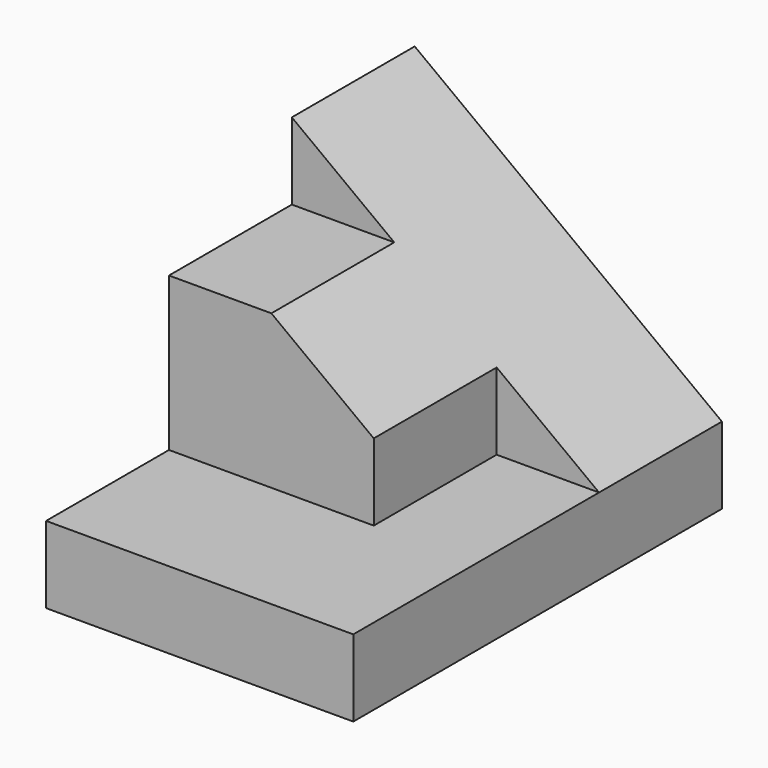
from build123d import *

# Parameters (mm, degrees)
F0_W     = 25.4
F0_H     = 6.35
F1_DEPTH = 38.1
F2_W     = 25.4
F2_H     = 6.35
F3_DEPTH = 25.401
F5_DEPTH = 25.4
F6_W     = 12.7
F6_H     = 6.35
F7_DEPTH = 25.401
F8_W     = 12.7
F8_H     = 6.35
F9_DEPTH = 25.401


# Not quite as in the source:
# - a feature names something its author has since deleted; it is built from what else it names


with BuildPart() as f1:
    # F0 (on Front) → F1 (new body)
    with BuildSketch(Plane.XZ):
        Polygon((25.4, 6.35), (0, 25.4), (0, 6.35), align=None)
        with Locations((12.7, 3.175)):
            Rectangle(F0_W, F0_H)
    extrude(amount=F1_DEPTH)

    # F2 (on face) → F3 (cut, through all)
    with BuildSketch(Plane(origin=(0, 0, 0), x_dir=(0, -1, 0), z_dir=(-1, 0, 0))):
        with Locations((25.4, 22.225)):
            Rectangle(F2_W, F2_H)
    extrude(amount=-F3_DEPTH, mode=Mode.SUBTRACT)

    # F4 (on face) → F5 (cut)
    with BuildSketch(Plane.XZ.offset(38.1)):
        Polygon((16.9333333333, 6.35), (25.4, 6.35), (16.9333333333, 12.7), align=None)
    extrude(amount=-F5_DEPTH, mode=Mode.SUBTRACT)

    # F6 (on face) → F7 (cut, through all)
    with BuildSketch(Plane(origin=(0, 0, 0), x_dir=(0, -1, 0), z_dir=(-1, 0, 0))):
        with Locations((31.75, 15.875)):
            Rectangle(F6_W, F6_H)
    extrude(amount=-F7_DEPTH, mode=Mode.SUBTRACT)

    # F8 (on face) → F9 (cut, through all)
    with BuildSketch(Plane(origin=(0, 0, 0), x_dir=(0, -1, 0), z_dir=(-1, 0, 0))):
        with Locations((31.75, 9.525)):
            Rectangle(F8_W, F8_H)
    extrude(amount=-F9_DEPTH, mode=Mode.SUBTRACT)


solid = f1.part
